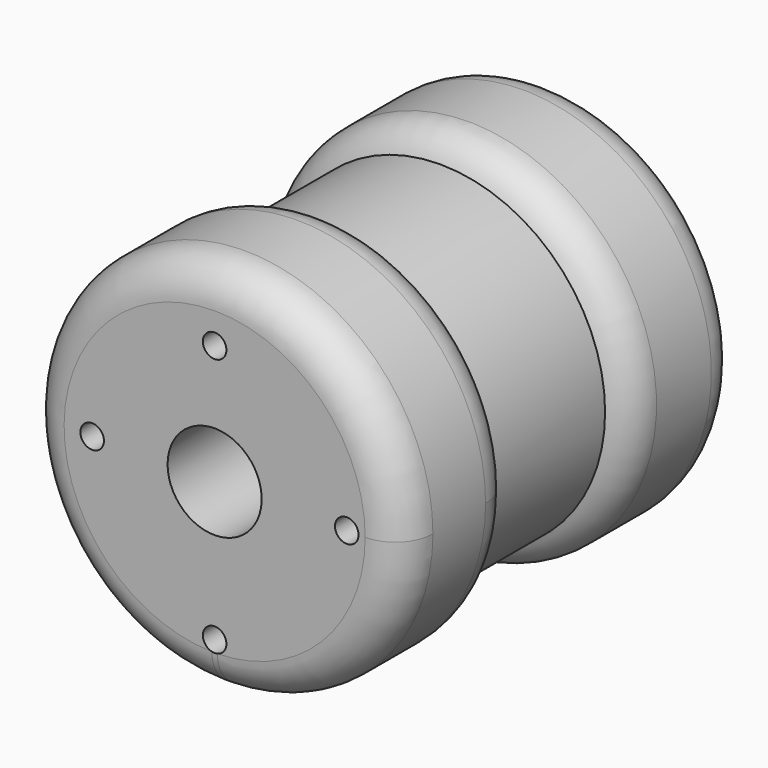
from build123d import *

# Parameters (mm, degrees)
F0_R      = 25.4
F1_DEPTH  = 19.05
F2_R      = 1.5875
F3_DEPTH  = 44.45
F4_R      = 5.08
F5_R      = 22.225
F6_DEPTH  = 19.05
F7_R      = 25.4
F8_DEPTH  = 19.05
F10_R     = 6.35
F11_DEPTH = 57.1510001


# Not quite as in the source:
# - a fillet or chamfer that OpenCascade refuses, or shapes differently, is made with other operations: its cross-section is extruded or revolved along the edge and cut away or added


with BuildPart() as f1:
    # F0 (on Front) → F1 (new body)
    with BuildSketch(Plane.XZ):
        Circle(F0_R)
    extrude(amount=F1_DEPTH)

    # F2 (on face) → F3 (cut)
    with BuildSketch(Plane(origin=(0, 0, 0), x_dir=(-1, 0, 0), z_dir=(0, 1, 0))):
        with Locations((0, 16.1551559669)):
            Circle(F2_R)
        with Locations((16.5286865403, 0)):
            Circle(F2_R)
        with Locations((0, -18.7698644697)):
            Circle(F2_R)
        with Locations((-17.8360380362, 0)):
            Circle(F2_R)
    extrude(amount=-F3_DEPTH, mode=Mode.SUBTRACT)

    # F4
    f4_edges = [f1.edges().sort_by_distance(p)[0] for p in [
        (-25.4, 0, 0),
        (-25.4, -19.05, 0),
    ]]
    fillet(f4_edges, radius=F4_R)

    # F5 (on Front) → F6 (join)
    with BuildSketch(Plane.XZ):
        Circle(F5_R)
    extrude(amount=-F6_DEPTH)

    # F7 (on face) → F8 (join)
    with BuildSketch(Plane(origin=(0, 19.05, 0), x_dir=(-1, 0, 0), z_dir=(0, 1, 0))):
        Circle(F7_R)
    extrude(amount=F8_DEPTH)

    # F9: fillet of radius 5.08 on 2 edges, made by hand

    # F9_s1 → F9_t2 (revolve, cut)
    with BuildSketch(Plane.XY):
        with BuildLine():
            ThreePointArc((-25.4, 33.02), (-23.9121024484, 36.6121024484), (-20.32, 38.1))
            Line((-20.32, 38.1), (-25.4, 38.1))
            Line((-25.4, 38.1), (-25.4, 33.02))
        make_face()
    revolve(axis=Axis((0, 38.1, 0), (0, 1, 0)), mode=Mode.SUBTRACT)

    # F9_s3 → F9_t4 (revolve, cut)
    with BuildSketch(Plane.XY):
        with BuildLine():
            ThreePointArc((-25.4, 23.7592860393), (-24.5321134838, 20.9194797079), (-22.225, 19.05))
            Line((-22.225, 19.05), (-25.4, 19.05))
            Line((-25.4, 19.05), (-25.4, 23.7592860393))
        make_face()
    revolve(axis=Axis((0, 19.05, 0), (0, 1, 0)), mode=Mode.SUBTRACT)

    # F10 (on face) → F11 (cut, through all)
    with BuildSketch(Plane(origin=(0, 38.1, 0), x_dir=(-1, 0, 0), z_dir=(0, 1, 0))):
        Circle(F10_R)
    extrude(amount=-F11_DEPTH, mode=Mode.SUBTRACT)


solid = f1.part
